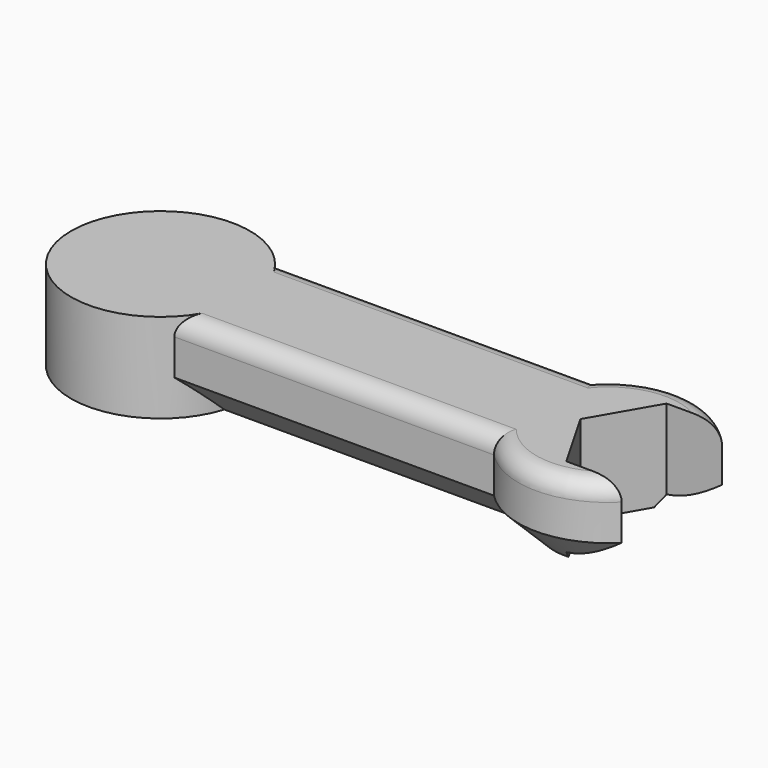
from build123d import *

# Parameters (mm, degrees)
F1_DEPTH = 6.35
F3_DEPTH = 12.701
F4_R     = 2.54
F5_SIZE  = 5.08


with BuildPart() as f1:
    # F0 (on Top) → F1 (new body, symmetric)
    with BuildSketch(Plane.XY):
        with BuildLine():
            Line((22.6803858958, 8.89), (-22.6803858958, 8.89))
            ThreePointArc((-22.6803858958, 8.89), (-44.45, 0), (-22.6803858958, -8.89))
            Line((-22.6803858958, -8.89), (22.6803858958, -8.89))
            ThreePointArc((22.6803858958, -8.89), (44.45, 0), (22.6803858958, 8.89))
        make_face()
    extrude(amount=F1_DEPTH, both=True)

    # F2 (on face) → F3 (cut, through all)
    with BuildSketch(Plane.XY.offset(6.35)):
        Polygon((27.8347122138, 0), (32.9673561069, -8.89), (43.2326438931, -8.89), (48.3652877862, 0), (43.2326438931, 8.89), (32.9673561069, 8.89), align=None)
    extrude(amount=-F3_DEPTH, mode=Mode.SUBTRACT)

    # F4
    f4_edges = [f1.edges().sort_by_distance(p)[0] for p in [
        (0, -8.89, 6.35),
        (31.75, -12.7, 6.35),
        (0, 8.89, 6.35),
        (31.75, 12.7, 6.35),
    ]]
    fillet(f4_edges, radius=F4_R)

    # F5
    f5_edges = [f1.edges().sort_by_distance(p)[0] for p in [
        (0, 8.89, -6.35),
        (31.75, 12.7, -6.35),
        (0, -8.89, -6.35),
        (31.75, -12.7, -6.35),
    ]]
    chamfer(f5_edges, length=F5_SIZE)


solid = f1.part
